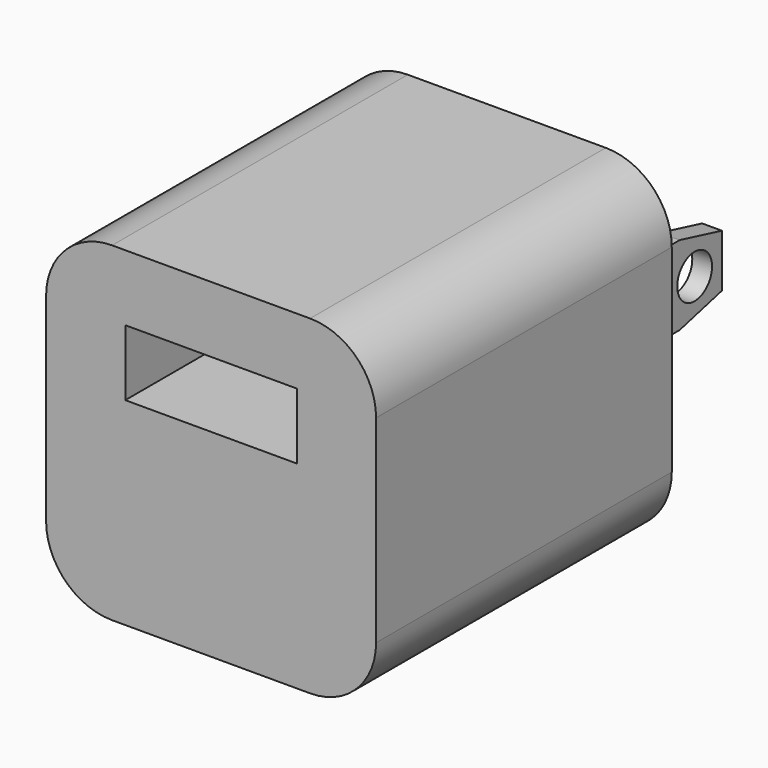
from build123d import *

# Parameters (mm, degrees)
F0_W      = 25
F0_H      = 25
F1_DEPTH  = 14
F3_DEPTH  = 15
F4_W      = 1.5
F4_H      = 6
F5_DEPTH  = 11
F6_R      = 1.65
F7_DEPTH  = 30.4
F8_R      = 5
F9_W      = 8.8653210551
F9_H      = 1.5135915019
F10_DEPTH = 10


with BuildPart() as f1:
    # F0 (on Front) → F1 (new body, symmetric)
    with BuildSketch(Plane.XZ):
        Rectangle(F0_W, F0_H)
    extrude(amount=F1_DEPTH, both=True)

    # F2 (on face) → F3 (cut)
    with BuildSketch(Plane.XZ.offset(14)):
        Polygon((-6.5, 2.5), (0, 2.5), (6.5, 2.5), (6.5, 7.5), (-6.5, 7.5), align=None)
    extrude(amount=-F3_DEPTH, mode=Mode.SUBTRACT)

    # F4 (on face) → F5 (join)
    with BuildSketch(Plane(origin=(0, 14, 0), x_dir=(-1, 0, 0), z_dir=(0, 1, 0))):
        with Locations((-6.75, 0.5)):
            Rectangle(F4_W, F4_H)
        with Locations((6.75, 0.5)):
            Rectangle(F4_W, F4_H)
    extrude(amount=F5_DEPTH)

    # F6 (on face) → F7 (cut)
    with BuildSketch(Plane.YZ.offset(7.5)):
        with Locations((22.4171727896, 0.5)):
            Circle(F6_R)
        Polygon((25, 2.4996667635), (25, 3.5), (21, 3.5), align=None)
        Polygon((25, -2.5), (25, -1.5), (21, -2.5), align=None)
    extrude(amount=-F7_DEPTH, mode=Mode.SUBTRACT)

    # F8
    f8_edges = [f1.edges().sort_by_distance(p)[0] for p in [
        (-12.5, 0, 12.5),
        (12.5, 0, 12.5),
        (12.5, 0, -12.5),
        (-12.5, 0, -12.5),
    ]]
    fillet(f8_edges, radius=F8_R)

    # F9 (on face) → F10 (join)
    with BuildSketch(Plane.XZ.offset(-1)):
        with Locations((0.1513590105, 5.6867792737)):
            Rectangle(F9_W, F9_H)
    extrude(amount=F10_DEPTH)


solid = f1.part
